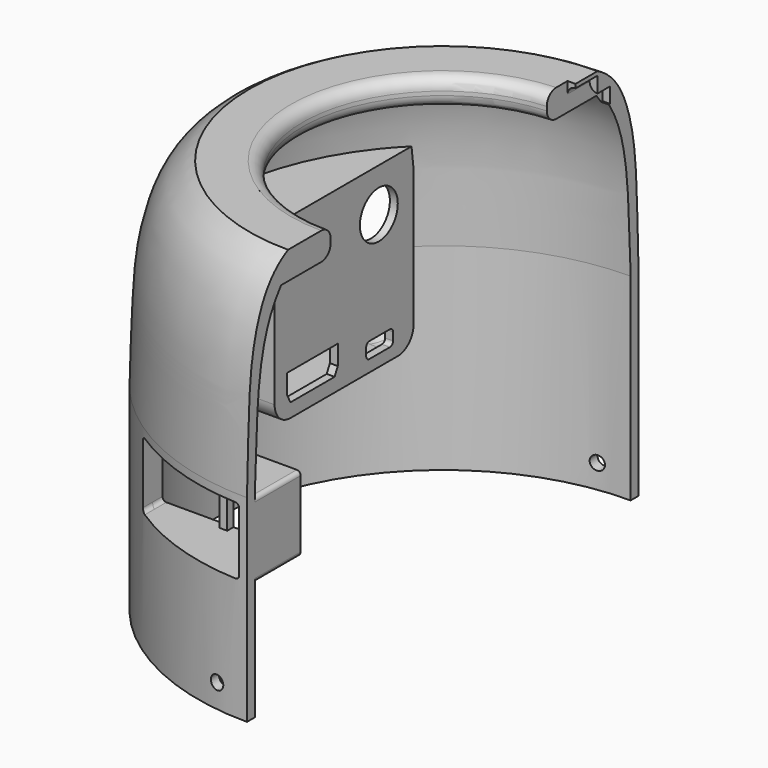
from build123d import *

# Parameters (mm, degrees)
F1_ANGLE_BACK = 90
F1_ANGLE      = 180
F3_DEPTH      = 49
F4_DEPTH      = 42
F5_DEPTH      = 53
F8_DEPTH      = 25
F9_END_RADIUS = 59.5
F9_REACH      = 83.9374760102
F10_DEPTH     = 2
F11_W         = 1
F11_H         = 5
F11_W_2       = 14
F11_H_2       = 2
F11_R         = 6
F12_DEPTH     = 2
F14_W         = 2
F14_H         = 17
F15_REACH     = 40.3462351599
F16_REACH     = 57.7072649741
F17_DEPTH     = 2
F18_R         = 1.75
F19_DEPTH     = 62.5


with BuildPart() as f1:
    # F0 (on Front) → F1 (revolve)
    with BuildSketch(Plane.XZ, mode=Mode.PRIVATE) as f1_sk:
        with BuildLine():
            ThreePointArc((-35.5, 47), (-36.3786796564, 49.1213203436), (-38.5, 50))
            Line((-38.5, 50), (-49, 50))
            add(Edge.make_bspline(
                [(-49, 50), (-50.0905438599, 49.4592544488), (-53.0493875637, 47.4989733534), (-57.4486951492, 41.931344871), (-61.5763053799, 28.0443008729), (-61.4881986154, 14.5014666819), (-62, 0)],
                knots=[0, 0, 0, 0, 0.1531073754, 0.3436852098, 0.6019385566, 1, 1, 1, 1], degree=3))
            Line((-62, 0), (-62, -50))
            Line((-62, -50), (-59.5, -50))
            Line((-59.5, -50), (-59.5, 0))
            add(Edge.make_bspline(
                [(-51.1955396277, 43), (-59.7999691963, 32.3488041759), (-58.4857873619, 15.5563373119), (-59.5, 0)],
                knots=[0, 0, 0, 0, 43.7945665817, 43.7945665817, 43.7945665817, 43.7945665817], degree=3))
            Line((-51.1955396277, 43), (-38.5, 43))
            ThreePointArc((-38.5, 43), (-36.3786796564, 43.8786796564), (-35.5, 46))
            Line((-35.5, 46), (-35.5, 47))
        make_face()
    revolve(f1_sk.sketch.rotate(Axis((0, 0, -47.5967168808), (0, 0, 1)), -F1_ANGLE_BACK), axis=Axis((0, 0, -47.5967168808), (0, 0, 1)), revolution_arc=F1_ANGLE)

    # F2 (on Front) → F3 (cut)
    with BuildSketch(Plane.XZ):
        with BuildLine():
            ThreePointArc((0, 45), (1.4142135624, 45.5857864376), (2, 47))
            ThreePointArc((2, 47), (1.4142135624, 48.4142135624), (0, 49))
            ThreePointArc((0, 49), (-1.3909130574, 48.4371363424), (-1.998931704, 47.0653608667))
            Line((-1.998931704, 47.0653608667), (-1.998931704, 46.9346391333))
            ThreePointArc((-1.998931704, 46.9346391333), (-1.3909130574, 45.5628636576), (0, 45))
        make_face()
    extrude(amount=-F3_DEPTH, mode=Mode.SUBTRACT)

    # F2 (on Front) → F4 (cut)
    with BuildSketch(Plane.XZ):
        with BuildLine():
            ThreePointArc((-1.998931704, 47.0653608667), (-1.3909130574, 48.4371363424), (0, 49))
            Line((0, 49), (0, 50.3604523001))
            Line((0, 50.3604523001), (-1.998931704, 50.3604523001))
            Line((-1.998931704, 50.3604523001), (-1.998931704, 47.0653608667))
        make_face()
    extrude(amount=-F4_DEPTH, mode=Mode.SUBTRACT)

    # F2 (on Front) → F5 (cut)
    with BuildSketch(Plane.XZ):
        with BuildLine():
            Line((0, 41.0653608667), (0, 45))
            ThreePointArc((0, 45), (-1.3909130574, 45.5628636576), (-1.998931704, 46.9346391333))
            Line((-1.998931704, 46.9346391333), (-1.998931704, 41.0653608667))
            Line((-1.998931704, 41.0653608667), (0, 41.0653608667))
        make_face()
    extrude(amount=-F5_DEPTH, mode=Mode.SUBTRACT)

    # F7 (on offset) → F8 (cut)
    with BuildSketch(Plane.YZ.offset(-41)):
        with BuildLine():
            Line((36, 22), (4, 22))
            ThreePointArc((4, 22), (0.4644660941, 20.5355339059), (-1, 17))
            Line((-1, 17), (-1, -16))
            ThreePointArc((-1, -16), (0.4644660941, -19.5355339059), (4, -21))
            Line((4, -21), (36, -21))
            ThreePointArc((36, -21), (39.5355339059, -19.5355339059), (41, -16))
            Line((41, -16), (41, 17))
            ThreePointArc((41, 17), (39.5355339059, 20.5355339059), (36, 22))
        make_face()
    extrude(amount=-F8_DEPTH, mode=Mode.SUBTRACT)

    f9_end = (Plane.XY.offset(-24.9999997) * Cylinder(F9_END_RADIUS, 509.7521236152, mode=Mode.PRIVATE)).faces().sort_by_distance((-59.5, 0, -24.9999997))[0]
    # F7 (on offset) → F9 (join, up to the whole of a round face its end follows)
    with BuildSketch(Plane.YZ.offset(-41)):
        with BuildLine():
            Line((42, -17), (42, 23))
            Line((42, 23), (-2, 23))
            Line((-2, 23), (-2, -17))
            ThreePointArc((-2, -17), (-0.5355339059, -20.5355339059), (3, -22))
            Line((3, -22), (37, -22))
            ThreePointArc((37, -22), (40.5355339059, -20.5355339059), (42, -17))
        make_face()
        with BuildLine():
            ThreePointArc((-1, 17), (0.4644660941, 20.5355339059), (4, 22))
            Line((4, 22), (36, 22))
            ThreePointArc((36, 22), (39.5355339059, 20.5355339059), (41, 17))
            Line((41, 17), (41, -16))
            ThreePointArc((41, -16), (39.5355339059, -19.5355339059), (36, -21))
            Line((36, -21), (4, -21))
            ThreePointArc((4, -21), (0.4644660941, -19.5355339059), (-1, -16))
            Line((-1, -16), (-1, 17))
        make_face(mode=Mode.SUBTRACT)
    f9_long = extrude(amount=-F9_REACH, mode=Mode.PRIVATE)
    add(split(f9_long, bisect_by=f9_end, keep=Keep.BOTTOM, mode=Mode.PRIVATE))

    # F7 (on offset) → F10 (join)
    with BuildSketch(Plane.YZ.offset(-41)):
        with BuildLine():
            Line((36, 22), (4, 22))
            ThreePointArc((4, 22), (0.4644660941, 20.5355339059), (-1, 17))
            Line((-1, 17), (-1, -16))
            ThreePointArc((-1, -16), (0.4644660941, -19.5355339059), (4, -21))
            Line((4, -21), (36, -21))
            ThreePointArc((36, -21), (39.5355339059, -19.5355339059), (41, -16))
            Line((41, -16), (41, 17))
            ThreePointArc((41, 17), (39.5355339059, 20.5355339059), (36, 22))
        make_face()
    extrude(amount=-F10_DEPTH)

    # F11 (on offset) → F12 (cut)
    with BuildSketch(Plane.YZ.offset(-41)):
        with BuildLine():
            Line((34.5, -15), (28, -15))
            ThreePointArc((28, -15), (27.2928932188, -15.2928932188), (27, -16))
            Line((27, -16), (27, -18))
            ThreePointArc((27, -18), (27.2928932188, -18.7071067812), (28, -19))
            Line((28, -19), (34.5, -19))
            ThreePointArc((34.5, -19), (35.2071067812, -18.7071067812), (35.5, -18))
            Line((35.5, -18), (35.5, -16))
            ThreePointArc((35.5, -16), (35.2071067812, -15.2928932188), (34.5, -15))
        make_face()
        with Locations((2.5, -14)):
            Rectangle(F11_W, F11_H)
        with Locations((10, -14)):
            Rectangle(F11_W_2, F11_H)
        Polygon((3, -16.5), (2, -16.5), (3, -18.5), align=None)
        with Locations((17.5, -14)):
            Rectangle(F11_W, F11_H)
        with Locations((10, -17.5)):
            Rectangle(F11_W_2, F11_H_2)
        Polygon((18, -16.5), (17, -16.5), (17, -18.5), align=None)
        with Locations((31, 12)):
            Circle(F11_R)
    extrude(amount=-F12_DEPTH, mode=Mode.SUBTRACT)

    f15_end = f1.faces().sort_by_distance((-62, 0, -24.9999997))[0]
    # F14 (on offset) → F15 (cut, up to a face of the model that its end follows)
    with BuildSketch(Plane.XZ.offset(45)):
        with Locations((-18, -10.5)):
            Rectangle(F14_W, F14_H)
        with BuildLine():
            Line((-19, -2), (-34, -2))
            ThreePointArc((-34, -2), (-34.7071067812, -2.2928932188), (-35, -3))
            Line((-35, -3), (-35, -18))
            ThreePointArc((-35, -18), (-34.7071067812, -18.7071067812), (-34, -19))
            Line((-34, -19), (-19, -19))
            Line((-19, -19), (-19, -2))
        make_face()
        with BuildLine():
            Line((-3, -2), (-17, -2))
            Line((-17, -2), (-17, -19))
            Line((-17, -19), (-3, -19))
            ThreePointArc((-3, -19), (-2.2928932188, -18.7071067812), (-2, -18))
            Line((-2, -18), (-2, -3))
            ThreePointArc((-2, -3), (-2.2928932188, -2.2928932188), (-3, -2))
        make_face()
    f15_long = extrude(amount=F15_REACH, mode=Mode.PRIVATE)
    add(split(f15_long, bisect_by=f15_end, keep=Keep.BOTTOM, mode=Mode.PRIVATE), mode=Mode.SUBTRACT)

    f16_end = f1.faces().sort_by_distance((-62, 0, -24.9999997))[0]
    # F14 (on offset) → F16 (join, up to a face of the model that its end follows)
    with BuildSketch(Plane.XZ.offset(45)):
        with BuildLine():
            ThreePointArc((0, -2), (-0.2928932188, -1.2928932188), (-1, -1))
            Line((-1, -1), (-35, -1))
            ThreePointArc((-35, -1), (-35.7071067812, -1.2928932188), (-36, -2))
            Line((-36, -2), (-36, -19))
            ThreePointArc((-36, -19), (-35.7071067812, -19.7071067812), (-35, -20))
            Line((-35, -20), (-1, -20))
            ThreePointArc((-1, -20), (-0.2928932188, -19.7071067812), (0, -19))
            Line((0, -19), (0, -2))
        make_face()
        with BuildLine():
            ThreePointArc((-35, -3), (-34.7071067812, -2.2928932188), (-34, -2))
            Line((-34, -2), (-19, -2))
            Line((-19, -2), (-17, -2))
            Line((-17, -2), (-3, -2))
            ThreePointArc((-3, -2), (-2.2928932188, -2.2928932188), (-2, -3))
            Line((-2, -3), (-2, -18))
            ThreePointArc((-2, -18), (-2.2928932188, -18.7071067812), (-3, -19))
            Line((-3, -19), (-17, -19))
            Line((-17, -19), (-19, -19))
            Line((-19, -19), (-34, -19))
            ThreePointArc((-34, -19), (-34.7071067812, -18.7071067812), (-35, -18))
            Line((-35, -18), (-35, -3))
        make_face(mode=Mode.SUBTRACT)
    f16_long = extrude(amount=F16_REACH, mode=Mode.PRIVATE)
    add(split(f16_long, bisect_by=f16_end, keep=Keep.ALL, mode=Mode.PRIVATE).solids().sort_by_distance((-0.4070626487, -45, -10.5))[0])

    # F14 (on offset) → F17 (join)
    with BuildSketch(Plane.XZ.offset(45)):
        with Locations((-18, -10.5)):
            Rectangle(F14_W, F14_H)
    extrude(amount=F17_DEPTH)

    # F18 (on Front) → F19 (cut, symmetric)
    with BuildSketch(Plane.XZ):
        with Locations((-8, -44)):
            Circle(F18_R)
    extrude(amount=F19_DEPTH, both=True, mode=Mode.SUBTRACT)


solid = f1.part
